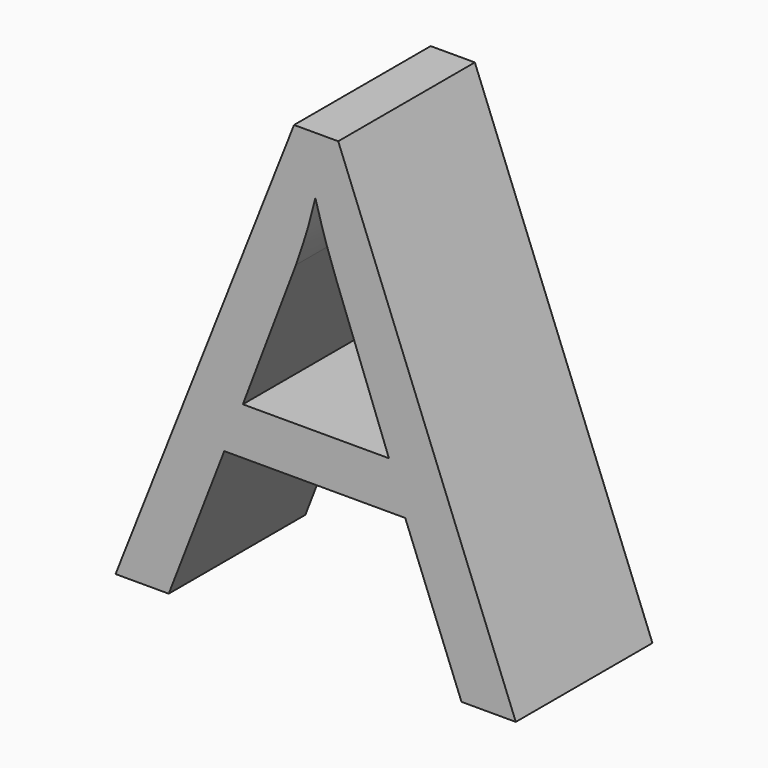
from build123d import *

# Parameters (mm, degrees)
F0_TEXT_SIZE = 70.5555555556
F1_DEPTH     = 19.05


# Not quite as in the source:
# - Text() gives the source's letters only with a copy of the font that has no kerning and outlines rounded to 1/6400 em; it was checked with that copy


with BuildPart() as f1:
    # F0 (on Front) → F1 (new body)
    with BuildSketch(Plane.XZ):
        with Locations((0, 0)):
            Text('A', F0_TEXT_SIZE, font='Open Sans', text_align=(TextAlign.LEFT, TextAlign.BOTTOM))
    extrude(amount=F1_DEPTH)


solid = f1.part
